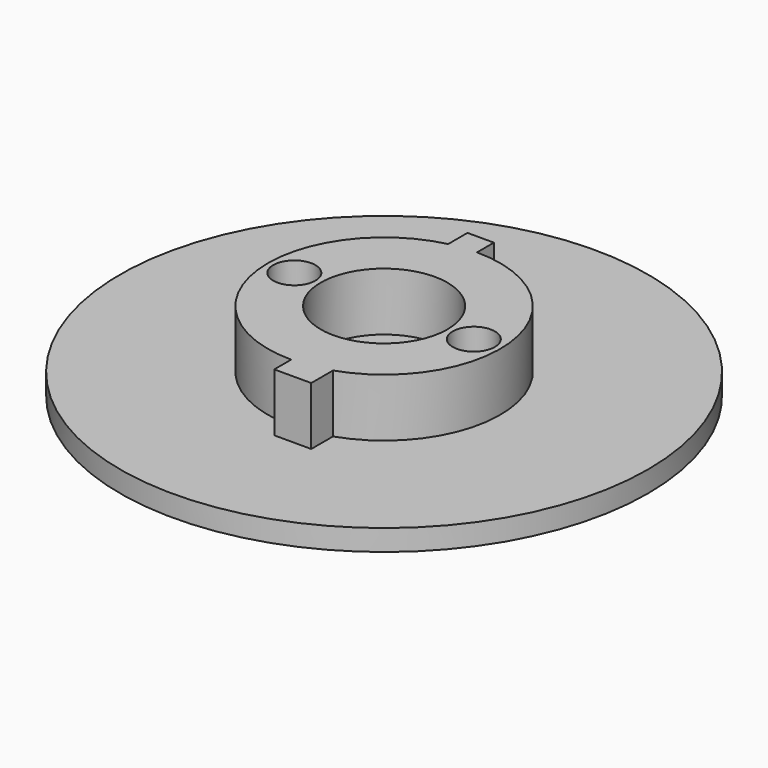
from build123d import *

# Parameters (mm, degrees)
F0_R           = 25
F0_R_2         = 6
F1_DEPTH       = 2
F2_DEPTH       = 7.5
F5_D           = 4
F5_CSINK_D     = 7
F5_CSINK_ANGLE = 90


# Not quite as in the source:
# - a feature names something its author has since deleted; it is built from what else it names


with BuildPart() as f1:
    # F0 (on Top) → F1 (new body)
    with BuildSketch(Plane.XY):
        Circle(F0_R)
        with BuildLine():
            ThreePointArc((0, 11), (7.7781745931, 7.7781745931), (11, 0))
            ThreePointArc((11, 0), (8.9302855497, -6.4226162893), (3.5, -10.4283268073))
            Line((3.5, -10.4283268073), (3.5, -13))
            Line((3.5, -13), (0, -13))
            Line((0, -13), (0, -11))
            ThreePointArc((0, -11), (-10.9277987049, -1.258258902), (-2.5, 10.7121426428))
            Line((-2.5, 10.7121426428), (-2.5, 13))
            Line((-2.5, 13), (0, 13))
            Line((0, 13), (0, 11))
        make_face(mode=Mode.SUBTRACT)
        with BuildLine():
            ThreePointArc((3.5, -10.4283268073), (8.9302855497, -6.4226162893), (11, 0))
            ThreePointArc((11, 0), (7.7781745931, 7.7781745931), (0, 11))
            ThreePointArc((0, 11), (-1.258258902, 10.9277987049), (-2.5, 10.7121426428))
            ThreePointArc((-2.5, 10.7121426428), (-10.9277987049, -1.258258902), (0, -11))
            ThreePointArc((0, -11), (1.773189939, -10.8561410013), (3.5, -10.4283268073))
        make_face()
        Circle(F0_R_2, mode=Mode.SUBTRACT)
        Circle(F0_R_2)
        with BuildLine():
            ThreePointArc((-2.5, 10.7121426428), (-1.258258902, 10.9277987049), (0, 11))
            Line((0, 11), (0, 13))
            Line((0, 13), (-2.5, 13))
            Line((-2.5, 13), (-2.5, 10.7121426428))
        make_face()
        with BuildLine():
            Line((3.5, -13), (3.5, -10.4283268073))
            ThreePointArc((3.5, -10.4283268073), (1.773189939, -10.8561410013), (0, -11))
            Line((0, -11), (0, -13))
            Line((0, -13), (3.5, -13))
        make_face()
    extrude(amount=F1_DEPTH)

    # F0 (on Top) → F2 (join)
    with BuildSketch(Plane.XY):
        with BuildLine():
            ThreePointArc((3.5, -10.4283268073), (8.9302855497, -6.4226162893), (11, 0))
            ThreePointArc((11, 0), (7.7781745931, 7.7781745931), (0, 11))
            ThreePointArc((0, 11), (-1.258258902, 10.9277987049), (-2.5, 10.7121426428))
            ThreePointArc((-2.5, 10.7121426428), (-10.9277987049, -1.258258902), (0, -11))
            ThreePointArc((0, -11), (1.773189939, -10.8561410013), (3.5, -10.4283268073))
        make_face()
        Circle(F0_R_2, mode=Mode.SUBTRACT)
        with BuildLine():
            Line((3.5, -13), (3.5, -10.4283268073))
            ThreePointArc((3.5, -10.4283268073), (1.773189939, -10.8561410013), (0, -11))
            Line((0, -11), (0, -13))
            Line((0, -13), (3.5, -13))
        make_face()
        with BuildLine():
            ThreePointArc((-2.5, 10.7121426428), (-1.258258902, 10.9277987049), (0, 11))
            Line((0, 11), (0, 13))
            Line((0, 13), (-2.5, 13))
            Line((-2.5, 13), (-2.5, 10.7121426428))
        make_face()
    extrude(amount=F2_DEPTH)

    # F5 (through all)
    with Locations(Plane(origin=(0, 0, 0), x_dir=(1, 0, 0), z_dir=(0, 0, -1))):
        with Locations((-8.5, 0), (8.5, 0)):
            CounterSinkHole(F5_D / 2, F5_CSINK_D / 2, counter_sink_angle=F5_CSINK_ANGLE)


solid = f1.part
